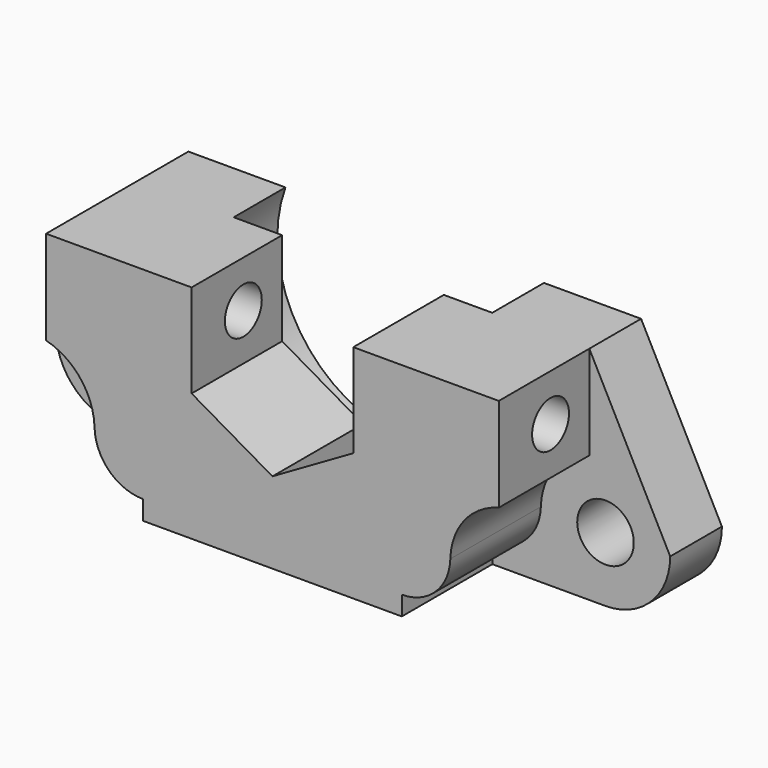
from build123d import *

# Parameters (mm, degrees)
F1_DEPTH = 7
F3_DEPTH = 34.2
F4_R     = 1.75
F5_DEPTH = 4
F6_R     = 4
F7_DEPTH = 25
F8_R     = 3
F9_DEPTH = 1.1867513459


with BuildPart() as f1:
    # F0 (on Front) → F1 (new body)
    with BuildSketch(Plane.XZ):
        Polygon((14, 2.8867513459), (5, 2.8867513459), (5, -2.8867513459), (0, -5.7735026919), (-5, -2.8867513459), (-5, 2.8867513459), (-14, 2.8867513459), (-14, -9.6132486541), (14, -9.6132486541), align=None)
    extrude(amount=F1_DEPTH)

    # F2 (on face) → F3 (cut)
    with BuildSketch(Plane.YZ.offset(14)):
        with BuildLine():
            ThreePointArc((-4.425, 0), (-3, -1.425), (-1.575, 0))
            Line((-1.575, 0), (-4.425, 0))
        make_face()
        with BuildLine():
            Line((-4.425, 0), (-1.575, 0))
            ThreePointArc((-1.575, 0), (-3, 1.425), (-4.425, 0))
        make_face()
    extrude(amount=-F3_DEPTH, mode=Mode.SUBTRACT)

    # F4 (on face) → F5 (join)
    with BuildSketch(Plane(origin=(0, 0, 0), x_dir=(-1, 0, 0), z_dir=(0, 1, 0))):
        with BuildLine():
            ThreePointArc((-5.1, -6.8), (-8.1441186755, -2.4337894321), (-7.9947899701, 2.8867513459))
            Line((-7.9947899701, 2.8867513459), (-14, 2.8867513459))
            Line((-14, 2.8867513459), (-19, -6.8))
            ThreePointArc((-19, -6.8), (-17.8284271247, -9.6284271247), (-15, -10.8))
            Line((-15, -10.8), (15, -10.8))
            ThreePointArc((15, -10.8), (17.8284271247, -9.6284271247), (19, -6.8))
            Line((19, -6.8), (14, 2.8867513459))
            Line((14, 2.8867513459), (7.9947899701, 2.8867513459))
            ThreePointArc((7.9947899701, 2.8867513459), (5.0550212811, -6.833502751), (-5.1, -6.8))
        make_face()
        with Locations((-15, -6.8)):
            Circle(F4_R, mode=Mode.SUBTRACT)
        with Locations((15, -6.8)):
            Circle(F4_R, mode=Mode.SUBTRACT)
    extrude(amount=F5_DEPTH)

    # F6 (on face) → F7 (cut)
    with BuildSketch(Plane.XZ):
        with Locations((-15, -6.8)):
            Circle(F6_R)
        with Locations((15, -6.8)):
            Circle(F6_R)
    extrude(amount=F7_DEPTH, mode=Mode.SUBTRACT)

    # F8
    f8_edges = [f1.edges().sort_by_distance(p)[0] for p in [
        (-12.156475, -3.5, -9.613249),
        (12.156475, -3.5, -9.613249),
    ]]
    fillet(f8_edges, radius=F8_R)

    # F9 (add, through all): a face of the model
    f9_faces = [f1.faces().sort_by_distance(p)[0] for p in [
        (0, -3.5, -9.6132486541),
    ]]
    extrude(f9_faces, amount=F9_DEPTH)


solid = f1.part
